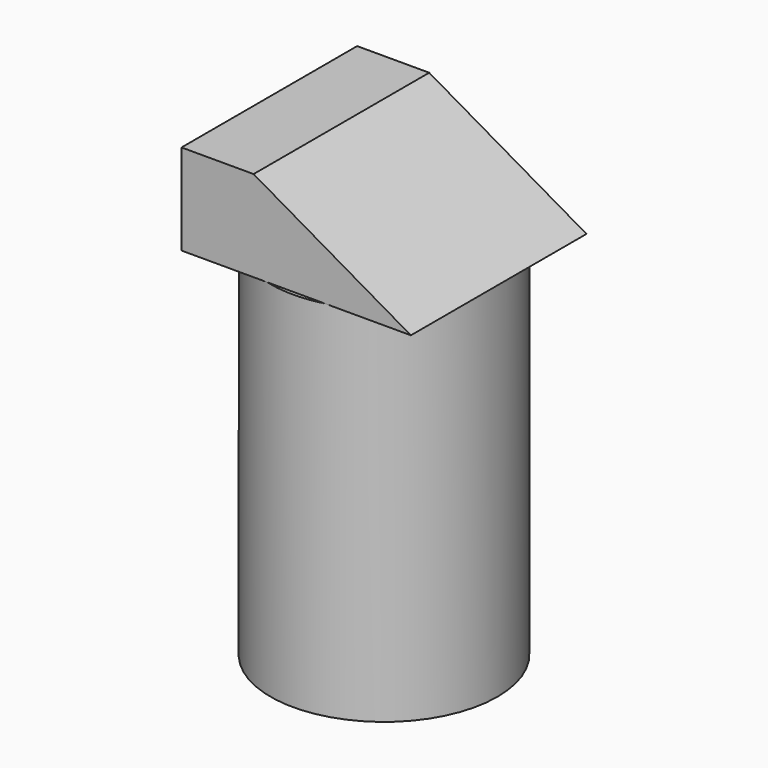
from build123d import *

# Parameters (mm, degrees)
F0_R     = 6.35
F1_DEPTH = 20.32
F2_W     = 12.8309261054
F2_H     = 12.2810313478
F3_DEPTH = 5.08
F4_SIZE2 = 8.798808
F4_SIZE  = 5.07999


# Not quite as in the source:
# - a fillet or chamfer is up to 0.001 mm smaller than in the source, because OpenCascade refuses the exact size


with BuildPart() as f1:
    # F0 (on Top) → F1 (new body)
    with BuildSketch(Plane.XY):
        Circle(F0_R)
    extrude(amount=F1_DEPTH)

    # F2 (on face) → F3 (join)
    with BuildSketch(Plane.XY.offset(20.32)):
        Rectangle(F2_W, F2_H)
    extrude(amount=F3_DEPTH)

    # F4 (size 5.08 and 8.7988181024 in the source; OpenCascade refuses exactly that, so slightly less here)
    f4_edges = [f1.edges().sort_by_distance(p)[0] for p in [
        (6.415463, 0, 25.4),
    ]]
    f4_side = f1.faces().sort_by_distance((6.415463, 0, 22.86))[0]
    chamfer(f4_edges, length=F4_SIZE, length2=F4_SIZE2, reference=f4_side)


solid = f1.part
